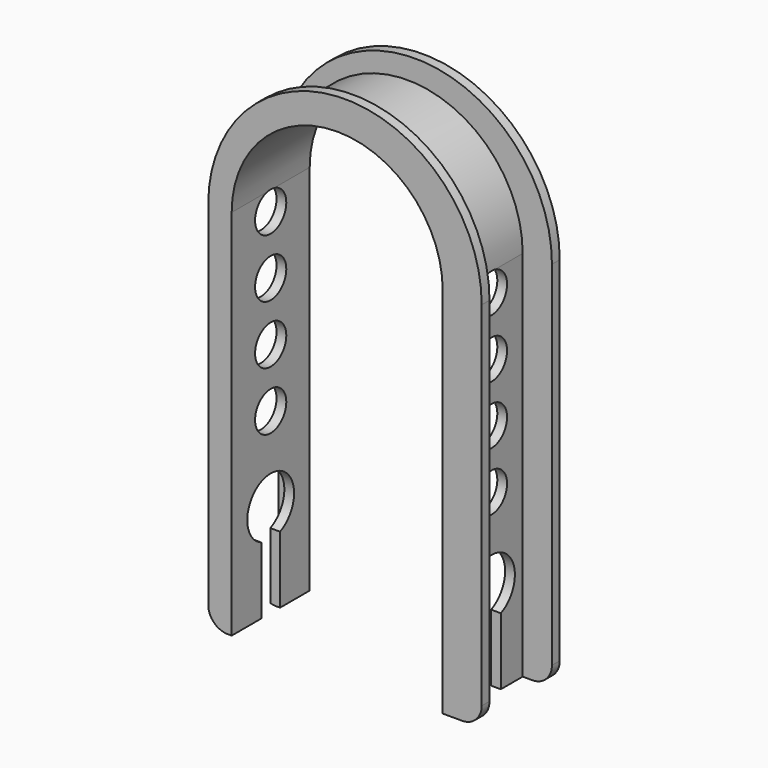
from build123d import *

# Parameters (mm, degrees)
F1_DEPTH  = 50
F2_T      = 5
F4_R      = 10
F5_DEPTH  = 125.1874270275
F6_DEPTH  = 125.1874270275
F7_W      = 40
F7_H      = 10
F8_DEPTH  = 15
F9_W      = 40
F9_H      = 10
F10_DEPTH = 7
F11_W     = 12
F11_H     = 5
F12_DEPTH = 125.1874270275


# Not quite as in the source:
# - a shell that OpenCascade refuses in one call is made with other operations: the cavity is built on its own and cut out
# - a feature names something its author has since deleted; it is built from what else it names


with BuildPart() as f1:
    # F0 (on Front) → F1 (new body)
    with BuildSketch(Plane.XZ):
        with BuildLine():
            Line((-68.1080648237, 65.760188823), (-68.1080648237, -115.239811177))
            ThreePointArc((-68.1080648237, -115.239811177), (-65.1791326356, -122.3108789889), (-58.1080648237, -125.239811177))
            Line((-58.1080648237, -125.239811177), (-56.1080648237, -125.239811177))
            Line((-56.1080648237, -125.239811177), (-56.1080648237, 65.760188823))
            ThreePointArc((-56.1080648237, 65.760188823), (-2.01485131, 119.8534023367), (52.0783622037, 65.760188823))
            Line((52.0783622037, 65.760188823), (52.0783622037, -125.239811177))
            Line((52.0783622037, -125.239811177), (62.0783622037, -125.239811177))
            ThreePointArc((62.0783622037, -125.239811177), (69.1494300156, -122.3108789889), (72.0783622037, -115.239811177))
            Line((72.0783622037, -115.239811177), (72.0783622037, 65.760188823))
            ThreePointArc((72.0783622037, 65.760188823), (1.98514869, 135.8534023367), (-68.1080648237, 65.760188823))
        make_face()
    extrude(amount=F1_DEPTH)

    # F2: shell of thickness 5, made by hand


with BuildPart() as f2_core1:
    # F2_t2: copy of F1
    add(f1.part)

    # the walls: a layer under each face that stays
    f2_faces = [f2_core1.faces().sort_by_distance(p)[0] for p in [
        (52.0783622037, -25, -29.739811177),
        (57.0783622037, -25, -125.239811177),
        (69.1494300156, -25, -122.3108789889),
        (-65.1791326356, -25, -122.3108789889),
        (-57.1080648237, -25, -125.239811177),
        (-56.1080648237, -25, -29.739811177),
        (-2.01485131, -25, 119.8534023367),
        (48.7139576992, 0, 92.3378667511),
        (48.7139576992, -50, 92.3378667511),
    ]]
    thicken(f2_faces, amount=-F2_T, mode=Mode.SUBTRACT)


with BuildPart() as f1_1:
    add(f1.part)

    # what is left inside the walls is the cavity
    f2_cavity = [f2_core1.part.solids().sort_by_distance(p)[0] for p in [
        (1.985149, -31.666667, 135.803402),
    ]]
    add(f2_cavity, mode=Mode.SUBTRACT)

    # F4 (on face) → F5 (cut, through all)
    with BuildSketch(Plane.YZ.offset(57.0783622037)):
        with Locations((-25, 55.9842178226)):
            Circle(F4_R)
        with Locations((-25, 25.9842178226)):
            Circle(F4_R)
        with Locations((-25, -4.0157821774)):
            Circle(F4_R)
        with Locations((-25, -34.0157821774)):
            Circle(F4_R)
    extrude(amount=-F5_DEPTH, mode=Mode.SUBTRACT)

    # F3 (on face) → F6 (cut, through all)
    with BuildSketch(Plane.YZ.offset(57.0783622037)):
        with BuildLine():
            Line((-19, -120.239811177), (-19, -90.9199170358))
            ThreePointArc((-19, -90.9199170358), (-25, -62.1721899509), (-31, -90.9199170358))
            Line((-31, -90.9199170358), (-31, -120.239811177))
            Line((-31, -120.239811177), (-19, -120.239811177))
        make_face()
    extrude(amount=-F6_DEPTH, mode=Mode.SUBTRACT)

    # F7 (on face) → F8 (cut)
    with BuildSketch(Plane.YZ.offset(72.0783622037)):
        with Locations((-25, -120.239811177)):
            Rectangle(F7_W, F7_H)
    extrude(amount=-F8_DEPTH, mode=Mode.SUBTRACT)

    # F9 (on face) → F10 (cut)
    with BuildSketch(Plane(origin=(-68.1080648237, 0, 0), x_dir=(0, -1, 0), z_dir=(-1, 0, 0))):
        with Locations((25, -120.239811177)):
            Rectangle(F9_W, F9_H)
    extrude(amount=-F10_DEPTH, mode=Mode.SUBTRACT)

    # F11 (on face) → F12 (cut, through all)
    with BuildSketch(Plane.YZ.offset(57.0783622037)):
        with Locations((-25, -122.739811177)):
            Rectangle(F11_W, F11_H)
    extrude(amount=-F12_DEPTH, mode=Mode.SUBTRACT)


solid = f1_1.part
